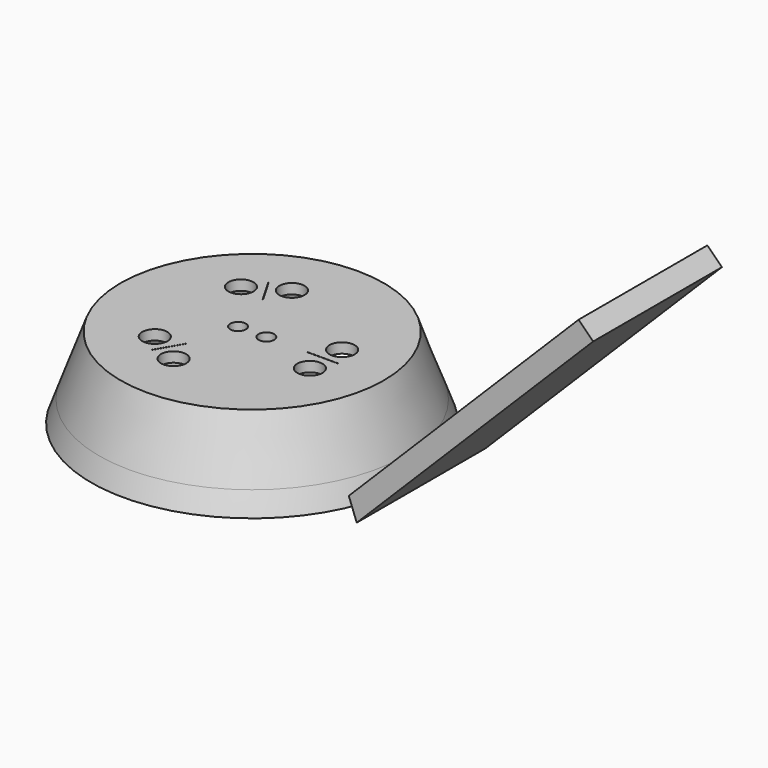
from build123d import *

# Parameters (mm, degrees)
F3_DEPTH      = 25.4
F3_DEPTH_BACK = 25.4
F4_T          = -3.175
F5_R          = 2.4673149282
F6_DEPTH      = 3.175
F7_R          = 3.96875
F8_DEPTH      = 3.175
F9_W          = 12.7
F9_H          = 3.3
F10_DEPTH     = 3.175
F11_W         = 9.5
F11_H         = 0.1
F12_DEPTH     = 25.4


# Not quite as in the source:
# - a feature names something its author has since deleted; it is built from what else it names


with BuildPart() as f1:
    # F0 (on Front) → F1 (revolve)
    with BuildSketch(Plane.XZ):
        Polygon((48.3660958283, 50.8), (41.5537999286, 69.5166291593), (0, 69.5166291593), (0, 53.5741299391), (0, 44.1166291593), (50.7986438789, 44.1166291593), align=None)
    revolve(axis=Axis((0, 0, 26.7870649695), (0, 0, -1)))

    # F4
    f4_openings = [f1.faces().sort_by_distance(p)[0] for p in [
        (0, 0, 44.116629),
    ]]
    offset(amount=F4_T, openings=f4_openings)

    # F5 (on face) → F6 (cut, through all)
    with BuildSketch(Plane.XY.offset(69.5166291593)):
        with Locations((-4.462592816, 0)):
            Circle(F5_R)
        with Locations((4.4704, 0)):
            Circle(F5_R)
    extrude(amount=-F6_DEPTH, mode=Mode.SUBTRACT)

    # F7 (on face) → F8 (cut, through all)
    with BuildSketch(Plane.XY.offset(69.5166291593)):
        with Locations((-6.1404809512, -23.3356249903)):
            Circle(F7_R)
        with Locations((-17.1390035792, -16.9856249903)):
            Circle(F7_R)
        with Locations((-17.1390035792, 16.9856249903)):
            Circle(F7_R)
        with Locations((-6.1404809512, 23.3356249903)):
            Circle(F7_R)
        with Locations((23.2794845304, 6.35)):
            Circle(F7_R)
        with Locations((23.2794845304, -6.35)):
            Circle(F7_R)
    extrude(amount=-F8_DEPTH, mode=Mode.SUBTRACT)

    # F9 (on face) → F10 (join)
    with BuildSketch(Plane(origin=(0, 0, 66.3416291593), x_dir=(1, 0, 0), z_dir=(0, 0, -1))):
        with Locations((22.225, 0)):
            Rectangle(F9_W, F9_H)
        Polygon((-6.5085580838, 14.5731532851), (-12.8585580838, 25.5716759131), (-15.7164419162, 23.9216759131), (-9.3664419162, 12.9231532851), align=None)
        Polygon((-9.3664419162, -12.9231532851), (-15.7164419162, -23.9216759131), (-12.8585580838, -25.5716759131), (-6.5085580838, -14.5731532851), align=None)
    extrude(amount=F10_DEPTH)

    # F11 (on face) → F12 (cut)
    with BuildSketch(Plane(origin=(0, 0, 63.1666291593), x_dir=(1, 0, 0), z_dir=(0, 0, -1))):
        with Locations((22.225, 0)):
            Rectangle(F11_W, F11_H)
        Polygon((-8.7808012702, -15.1087939311), (-13.5308012702, -23.3360352671), (-13.4441987298, -23.3860352671), (-8.6941987298, -15.1587939311), align=None)
        Polygon((-8.6941987298, 15.1587939311), (-13.4441987298, 23.3860352671), (-13.5308012702, 23.3360352671), (-8.7808012702, 15.1087939311), align=None)
    extrude(amount=-F12_DEPTH, mode=Mode.SUBTRACT)


with BuildPart() as f3:
    # F2 (on Front) → F3 (new body, two sides)
    with BuildSketch(Plane.XZ) as f3_sk:
        Polygon((53.2972933905, 44.1405509586), (127.8775462373, 118.7208038053), (123.2991750213, 123.2991750213), (50.8, 50.8), align=None)
    extrude(amount=F3_DEPTH)
    extrude(f3_sk.sketch, amount=-F3_DEPTH_BACK)


solid = Compound([f1.part, f3.part])
